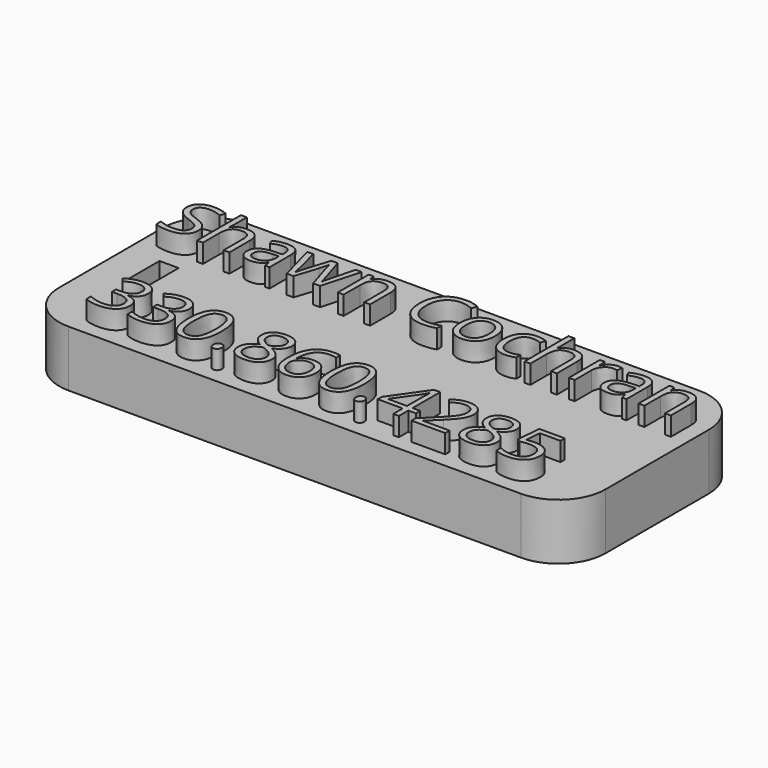
from build123d import *

# Parameters (mm, degrees)
F0_W         = 58.2218244672
F0_H         = 23.7748990767
F1_DEPTH     = 6
F2_R         = 5
F5_TEXT_SIZE = 7.6717528657
F4_TEXT_SIZE = 7.6998040353
F6_DEPTH     = 2
F7_W         = 2.0408891141
F7_H         = 4.1555203497
F8_DEPTH     = 6


# Not quite as in the source:
# - Text() gives the source's letters only with a copy of the font that has no kerning and outlines rounded to 1/6400 em; it was checked with that copy


with BuildPart() as f1:
    # F0 (on Top) → F1 (new body)
    with BuildSketch(Plane.XY):
        Rectangle(F0_W, F0_H)
    extrude(amount=F1_DEPTH)

    # F2
    f2_edges = [f1.edges().sort_by_distance(p)[0] for p in [
        (-29.110912, 11.88745, 3),
        (29.110912, 11.88745, 3),
        (29.110912, -11.88745, 3),
        (-29.110912, -11.88745, 3),
    ]]
    fillet(f2_edges, radius=F2_R)

    # F5 (on face) + F4 (on face) → F6 (join)
    with BuildSketch(Plane.XY.offset(6)):
        with Locations((-24, -10.2935134303)):
            Text('330.860.4285', F5_TEXT_SIZE, font='Open Sans', text_align=(TextAlign.LEFT, TextAlign.BOTTOM))
    with BuildSketch(Plane.XY.offset(6)):
        with Locations((-27.9406638931, 3.913574458)):
            Text('Shawn Cochran', F4_TEXT_SIZE, font='Open Sans', text_align=(TextAlign.LEFT, TextAlign.BOTTOM))
    extrude(amount=F6_DEPTH)

    # F7 (on face) → F8 (cut, through all)
    with BuildSketch(Plane.XY.offset(6)):
        with Locations((-24.5690140873, 0)):
            Rectangle(F7_W, F7_H)
    extrude(amount=-F8_DEPTH, mode=Mode.SUBTRACT)


solid = f1.part
